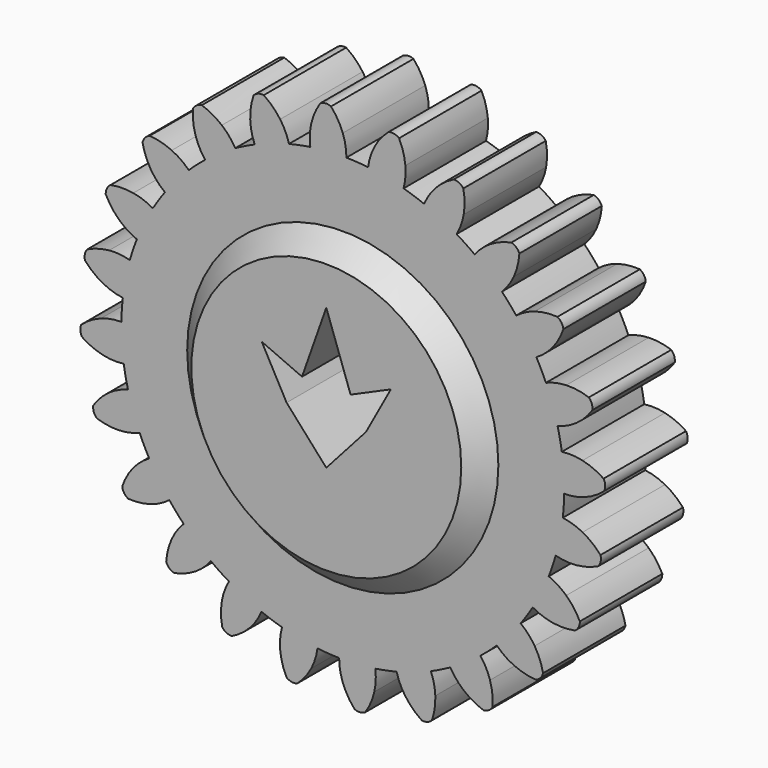
from build123d import *

# Parameters (mm, degrees)
F0_R     = 37.7460483738
F1_DEPTH = 25
F2_COUNT = 24
F3_DEPTH = 30
F4_SIZE  = 4.99999


# Not quite as in the source:
# - a fillet or chamfer is up to 0.001 mm smaller than in the source, because OpenCascade refuses the exact size


with BuildPart() as f1:
    # F0 (on Front) → F1 (new body)
    with BuildSketch(Plane.XZ):
        with BuildLine():
            ThreePointArc((-7.8842675869, 53.139290225), (-3.5135215054, 53.6059792153), (0.8807473744, 53.7137796572))
            ThreePointArc((0.8807473744, 53.7137796572), (0.6630516081, 56.2334289984), (0, 58.674))
            ThreePointArc((0, 58.674), (-1.206752041, 61.1877140894), (-2.8564405638, 63.4357213824))
            ThreePointArc((-2.8564405638, 63.4357213824), (-4.1730505874, 63.6684485091), (-5.448019844, 63.2658603022))
            ThreePointArc((-5.448019844, 63.2658603022), (-6.7901712207, 60.821757462), (-7.6584938023, 58.1720357962))
            ThreePointArc((-7.6584938023, 58.1720357962), (-7.9973144723, 55.6657986162), (-7.8842675869, 53.139290225))
        make_face()
        with BuildLine():
            ThreePointArc((-7.8842675869, 53.139290225), (-35.0884247435, -40.6785974441), (53.721, 0))
            ThreePointArc((53.721, 0), (38.2966086664, 37.6738052983), (0.8807473744, 53.7137796572))
            ThreePointArc((0.8807473744, 53.7137796572), (-3.5135215054, 53.6059792153), (-7.8842675869, 53.139290225))
        make_face()
        Circle(F0_R, mode=Mode.SUBTRACT)
    extrude(amount=F1_DEPTH)


with BuildPart() as f2_1:
    # F2: instance of F1
    add(f1.part.rotate(Axis((0, 0, 0), (0, 1, 0)), 1 * 360 / F2_COUNT))


with BuildPart() as f2_2:
    # F2: instance of F1
    add(f1.part.rotate(Axis((0, 0, 0), (0, 1, 0)), 2 * 360 / F2_COUNT))


with BuildPart() as f2_3:
    # F2: instance of F1
    add(f1.part.rotate(Axis((0, 0, 0), (0, 1, 0)), 3 * 360 / F2_COUNT))


with BuildPart() as f2_4:
    # F2: instance of F1
    add(f1.part.rotate(Axis((0, 0, 0), (0, 1, 0)), 4 * 360 / F2_COUNT))


with BuildPart() as f2_5:
    # F2: instance of F1
    add(f1.part.rotate(Axis((0, 0, 0), (0, 1, 0)), 5 * 360 / F2_COUNT))


with BuildPart() as f2_6:
    # F2: instance of F1
    add(f1.part.rotate(Axis((0, 0, 0), (0, 1, 0)), 6 * 360 / F2_COUNT))


with BuildPart() as f2_7:
    # F2: instance of F1
    add(f1.part.rotate(Axis((0, 0, 0), (0, 1, 0)), 7 * 360 / F2_COUNT))


with BuildPart() as f2_8:
    # F2: instance of F1
    add(f1.part.rotate(Axis((0, 0, 0), (0, 1, 0)), 8 * 360 / F2_COUNT))


with BuildPart() as f2_9:
    # F2: instance of F1
    add(f1.part.rotate(Axis((0, 0, 0), (0, 1, 0)), 9 * 360 / F2_COUNT))


with BuildPart() as f2_10:
    # F2: instance of F1
    add(f1.part.rotate(Axis((0, 0, 0), (0, 1, 0)), 10 * 360 / F2_COUNT))


with BuildPart() as f2_11:
    # F2: instance of F1
    add(f1.part.rotate(Axis((0, 0, 0), (0, 1, 0)), 11 * 360 / F2_COUNT))


with BuildPart() as f2_12:
    # F2: instance of F1
    add(f1.part.rotate(Axis((0, 0, 0), (0, 1, 0)), 12 * 360 / F2_COUNT))


with BuildPart() as f2_13:
    # F2: instance of F1
    add(f1.part.rotate(Axis((0, 0, 0), (0, 1, 0)), 13 * 360 / F2_COUNT))


with BuildPart() as f2_14:
    # F2: instance of F1
    add(f1.part.rotate(Axis((0, 0, 0), (0, 1, 0)), 14 * 360 / F2_COUNT))


with BuildPart() as f2_15:
    # F2: instance of F1
    add(f1.part.rotate(Axis((0, 0, 0), (0, 1, 0)), 15 * 360 / F2_COUNT))


with BuildPart() as f2_16:
    # F2: instance of F1
    add(f1.part.rotate(Axis((0, 0, 0), (0, 1, 0)), 16 * 360 / F2_COUNT))


with BuildPart() as f2_17:
    # F2: instance of F1
    add(f1.part.rotate(Axis((0, 0, 0), (0, 1, 0)), 17 * 360 / F2_COUNT))


with BuildPart() as f2_18:
    # F2: instance of F1
    add(f1.part.rotate(Axis((0, 0, 0), (0, 1, 0)), 18 * 360 / F2_COUNT))


with BuildPart() as f2_19:
    # F2: instance of F1
    add(f1.part.rotate(Axis((0, 0, 0), (0, 1, 0)), 19 * 360 / F2_COUNT))


with BuildPart() as f2_20:
    # F2: instance of F1
    add(f1.part.rotate(Axis((0, 0, 0), (0, 1, 0)), 20 * 360 / F2_COUNT))


with BuildPart() as f2_21:
    # F2: instance of F1
    add(f1.part.rotate(Axis((0, 0, 0), (0, 1, 0)), 21 * 360 / F2_COUNT))


with BuildPart() as f2_22:
    # F2: instance of F1
    add(f1.part.rotate(Axis((0, 0, 0), (0, 1, 0)), 22 * 360 / F2_COUNT))


with BuildPart() as f2_23:
    # F2: instance of F1
    add(f1.part.rotate(Axis((0, 0, 0), (0, 1, 0)), 23 * 360 / F2_COUNT))


with BuildPart() as f1_1:
    add(f1.part)

    add(f2_1.part)  # F3 merges F2_1

    add(f2_2.part)  # F3 merges F2_2

    add(f2_3.part)  # F3 merges F2_3

    add(f2_4.part)  # F3 merges F2_4

    add(f2_5.part)  # F3 merges F2_5

    add(f2_6.part)  # F3 merges F2_6

    add(f2_7.part)  # F3 merges F2_7

    add(f2_8.part)  # F3 merges F2_8

    add(f2_9.part)  # F3 merges F2_9

    add(f2_10.part)  # F3 merges F2_10

    add(f2_11.part)  # F3 merges F2_11

    add(f2_12.part)  # F3 merges F2_12

    add(f2_13.part)  # F3 merges F2_13

    add(f2_14.part)  # F3 merges F2_14

    add(f2_15.part)  # F3 merges F2_15

    add(f2_16.part)  # F3 merges F2_16

    add(f2_17.part)  # F3 merges F2_17

    add(f2_18.part)  # F3 merges F2_18

    add(f2_19.part)  # F3 merges F2_19

    add(f2_20.part)  # F3 merges F2_20

    add(f2_21.part)  # F3 merges F2_21

    add(f2_22.part)  # F3 merges F2_22

    add(f2_23.part)  # F3 merges F2_23
    # F0 (on Front) → F3 (join)
    with BuildSketch(Plane.XZ):
        Circle(F0_R)
        Polygon((0, -10.7778282836), (-9.6281943843, 0), (-15.6637784094, 11.0652372241), (-5.8918795548, 6.7541059107), (0, 23.4238151461), (5.8918795548, 6.7541059107), (15.6637784094, 11.0652372241), (9.6281943843, 0), align=None, mode=Mode.SUBTRACT)
    extrude(amount=F3_DEPTH)

    # F4 (size 5 in the source; OpenCascade refuses exactly that, so slightly less here)
    f4_edges = [f1_1.edges().sort_by_distance(p)[0] for p in [
        (-37.746048, -30, 0),
    ]]
    chamfer(f4_edges, length=F4_SIZE)


solid = f1_1.part
